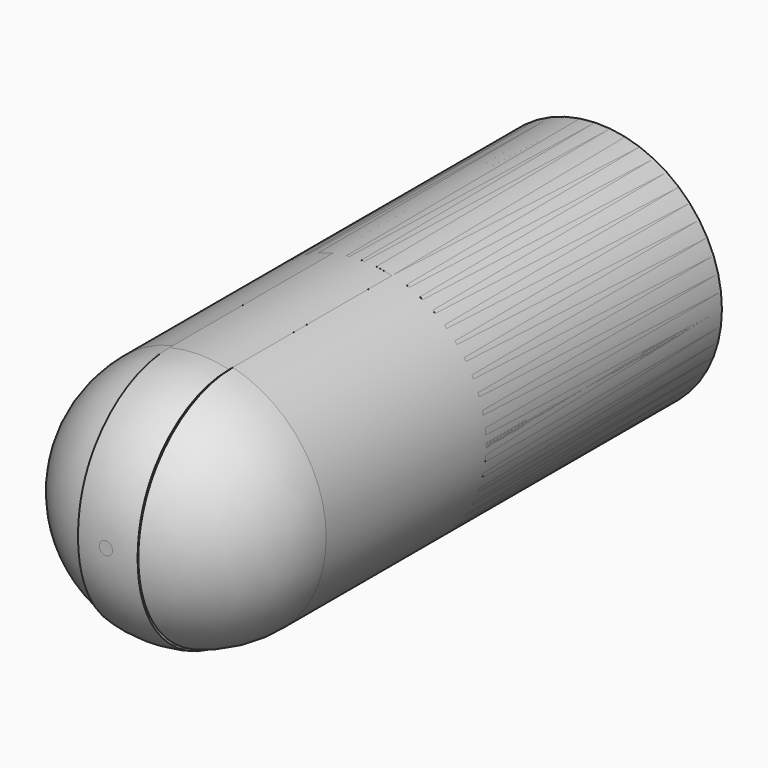
from build123d import *

# Parameters (mm, degrees)
F0_R      = 6.35
F1_DEPTH  = 31.75
F2_R      = 6.2547444974
F3_W      = 1.5368231577
F3_H      = 10.16
F4_DEPTH  = 23.1394
F5_R      = 2.2298122128
F6_DEPTH  = 2.5146
F8_DEPTH  = 31.75
F9_R      = 6.0094603995
F7_W      = 7.8039629152
F7_H      = 20.3567193821
F10_DEPTH = 12.7
F11_R     = 3.2850641109
F12_DEPTH = 19.2278


# Not quite as in the source:
# - a feature names something its author has since deleted; it is built from what else it names


with BuildPart() as f1:
    # F0 (on Front) → F1 (new body)
    with BuildSketch(Plane.XZ):
        Circle(F0_R)
    extrude(amount=F1_DEPTH)

    # F2
    f2_edges = [f1.edges().sort_by_distance(p)[0] for p in [
        (-6.35, -31.75, 0),
    ]]
    fillet(f2_edges, radius=F2_R)

    # F3 (on Top) → F4 (cut, symmetric)
    with BuildSketch(Plane.XY):
        with Locations((-0.7684115789, -30.4810036588)):
            Rectangle(F3_W, F3_H)
        with Locations((0.7684115789, -30.4810036588)):
            Rectangle(F3_W, F3_H)
        with Locations((0.7684115789, -20.3210036588)):
            Rectangle(F3_W, F3_H)
        with Locations((-0.7684115789, -20.3210036588)):
            Rectangle(F3_W, F3_H)
    extrude(amount=F4_DEPTH, both=True, mode=Mode.SUBTRACT)

    # F5 (on Right) → F6 (join, symmetric)
    with BuildSketch(Plane.YZ):
        with Locations((-25.498393923, 0)):
            Circle(F5_R)
    extrude(amount=F6_DEPTH, both=True)


with BuildPart() as f8:
    # F0 (on Front) → F8 (new body)
    with BuildSketch(Plane.XZ):
        Circle(F0_R)
    extrude(amount=F8_DEPTH)

    # F9
    f9_edges = [f8.edges().sort_by_distance(p)[0] for p in [
        (-6.35, -31.75, 0),
    ]]
    fillet(f9_edges, radius=F9_R)

    # F7 (on Top) → F10 (cut, symmetric)
    with BuildSketch(Plane.XY):
        with Locations((-5.43864473, -25.3729536198)):
            Rectangle(F7_W, F7_H)
        with Locations((5.43864473, -25.3729536198)):
            Rectangle(F7_W, F7_H)
    extrude(amount=F10_DEPTH, both=True, mode=Mode.SUBTRACT)

    # F11 (on Right) → F12 (cut, symmetric)
    with BuildSketch(Plane.YZ):
        with Locations((-25.3563765436, 0)):
            Circle(F11_R)
    extrude(amount=F12_DEPTH, both=True, mode=Mode.SUBTRACT)


solid = Compound([f1.part, f8.part])
